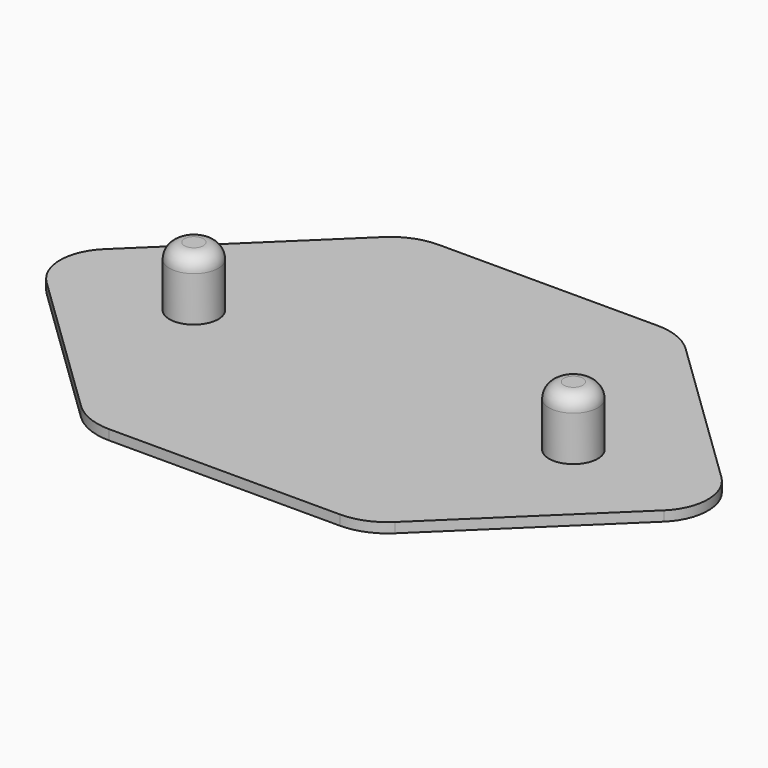
from build123d import *

# Parameters (mm, degrees)
F0_R     = 2.45
F1_DEPTH = 1
F2_DEPTH = 6
F3_R     = 1.5
F4_R     = 1.5
F5_DEPTH = 1


# Not quite as in the source:
# - a feature names something its author has since deleted; it is built from what else it names


with BuildPart() as f1:
    # F0 (on Top) → F1 (new body)
    with BuildSketch(Plane.XY):
        with BuildLine():
            Line((10.9931575138, 20.5618447948), (0, 20.5618447948))
            Line((0, 20.5618447948), (0, -20))
            Line((0, -20), (11.5745256156, -20))
            ThreePointArc((11.5745256156, -20), (13.8232148234, -19.5626789272), (15.7441043055, -18.3144656157))
            Line((15.7441043055, -18.3144656157), (30.9746489082, -3.5953880131))
            ThreePointArc((30.9746489082, -3.5953880131), (32.5, 0), (30.9746489082, 3.5953880131))
            Line((30.9746489082, 3.5953880131), (15.1627362037, 18.8763104104))
            ThreePointArc((15.1627362037, 18.8763104104), (13.2418467215, 20.124523722), (10.9931575138, 20.5618447948))
        make_face()
        with Locations((19, 0)):
            Circle(F0_R, mode=Mode.SUBTRACT)
        with BuildLine():
            Line((0, 20.5618447948), (-10.9931575138, 20.5618447948))
            ThreePointArc((-10.9931575138, 20.5618447948), (-13.2418467215, 20.124523722), (-15.1627362037, 18.8763104104))
            Line((-15.1627362037, 18.8763104104), (-30.9746489082, 3.5953880131))
            ThreePointArc((-30.9746489082, 3.5953880131), (-32.5, 0), (-30.9746489082, -3.5953880131))
            Line((-30.9746489082, -3.5953880131), (-15.7441043055, -18.3144656157))
            ThreePointArc((-15.7441043055, -18.3144656157), (-13.8232148234, -19.5626789272), (-11.5745256156, -20))
            Line((-11.5745256156, -20), (0, -20))
            Line((0, -20), (0, 20.5618447948))
        make_face()
        with Locations((-19, -0.0933343646)):
            Circle(F0_R, mode=Mode.SUBTRACT)
    extrude(amount=-F1_DEPTH)


with BuildPart() as f2:
    # F0 (on Top) → F2 (new body)
    with BuildSketch(Plane.XY):
        with Locations((-19, -0.0933343646)):
            Circle(F0_R)
    extrude(amount=F2_DEPTH)

    # F3
    f3_edges = [f2.edges().sort_by_distance(p)[0] for p in [
        (-21.45, -0.093334, 6),
    ]]
    fillet(f3_edges, radius=F3_R)


with BuildPart() as f2b:
    # F0 (on Top) → F2, piece 2 (new body)
    with BuildSketch(Plane.XY):
        with Locations((19, 0)):
            Circle(F0_R)
    extrude(amount=F2_DEPTH)

    # F4
    f4_edges = [f2b.edges().sort_by_distance(p)[0] for p in [
        (16.55, 0, 6),
    ]]
    fillet(f4_edges, radius=F4_R)


with BuildPart() as f5:
    # F5 (new): a face of the model
    f5_faces = [f2b.part.faces().sort_by_distance(p)[0] for p in [
        (19, 0, 0),
    ]]
    extrude(f5_faces, amount=F5_DEPTH)


with BuildPart() as f5b:
    # F5#2 (new): a face of the model
    f5_2_faces = [f2.part.faces().sort_by_distance(p)[0] for p in [
        (-19, -0.0933343646, 0),
    ]]
    extrude(f5_2_faces, amount=F5_DEPTH)


solid = Compound([f1.part, f2.part, f2b.part, f5.part, f5b.part])
